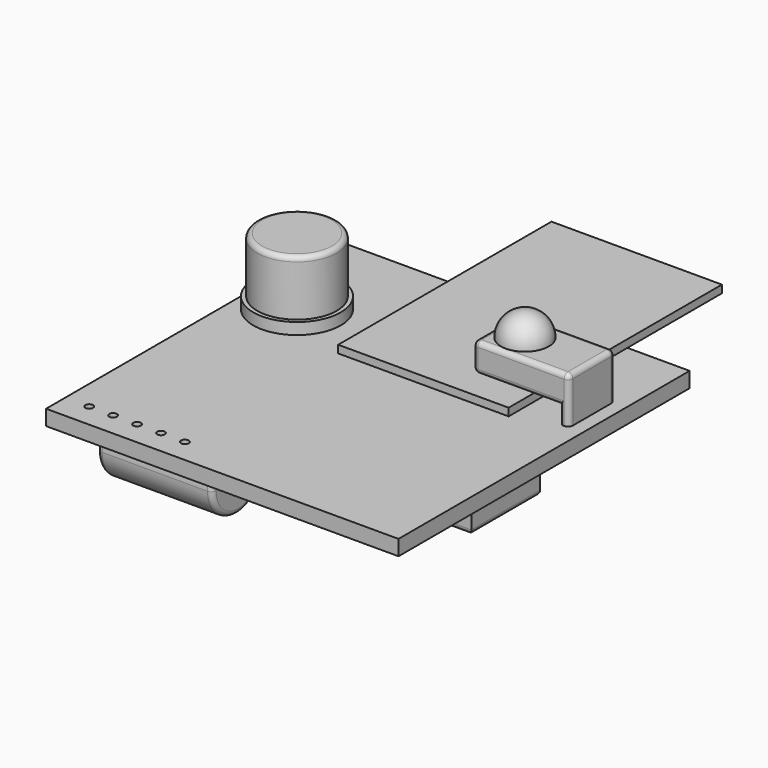
from build123d import *

# Parameters (mm, degrees)
F0_R      = 4.15
F0_W      = 10
F0_H      = 6
F1_DEPTH  = 1.6
F2_R      = 4.575
F2_R_2    = 4.15
F3_DEPTH  = 1.2
F4_R      = 4.15
F5_DEPTH  = 5.8
F2_W      = 4.9
F2_H      = 6
F2_W_2    = 17.8
F2_H_2    = 12.34
F6_DEPTH  = 0.8
F9_W      = 1
F9_H      = 6
F10_DEPTH = 1.8
F8_W      = 10
F8_H      = 6
F11_DEPTH = 3
F12_R     = 2.5
F13_DEPTH = 2.5
F14_R     = 2.49999
F15_R     = 0.49999
F16_R     = 0.4
F17_DEPTH = 25
F20_DEPTH = 12
F21_R     = 0.5
F22_W     = 18
F22_H     = 9
F23_DEPTH = 2.6
F24_R     = 0.5


# Not quite as in the source:
# - a fillet or chamfer is up to 0.001 mm smaller than in the source, because OpenCascade refuses the exact size


with BuildPart() as f1:
    # F0 (on Top) → F1 (new body)
    with BuildSketch(Plane.XY):
        Polygon((-25.5229242146, 29.8087272195), (-38.0229242146, 29.8087272195), (-38.0229242146, -8.1912727805), (-1.2229242146, -8.1912727805), (-1.2229242146, 29.8087272195), (-7.7229242146, 29.8087272195), align=None)
        with Locations((-33.0229242146, 18.3087272195)):
            Circle(F0_R, mode=Mode.SUBTRACT)
        with Locations((-7.6229242146, 18.8087272195)):
            Rectangle(F0_W, F0_H, mode=Mode.SUBTRACT)
        with Locations((-33.0229242146, 18.3087272195)):
            Circle(F0_R)
        with Locations((-7.6229242146, 18.8087272195)):
            Rectangle(F0_W, F0_H)
    extrude(amount=-F1_DEPTH)

    # F2 (on face) → F3 (join)
    with BuildSketch(Plane.XY):
        with Locations((-33.0229242146, 18.3087272195)):
            Circle(F2_R)
        with Locations((-33.0229242146, 18.3087272195)):
            Circle(F2_R_2, mode=Mode.SUBTRACT)
        with Locations((-33.0229242146, 18.3087272195)):
            Circle(F2_R_2)
    extrude(amount=F3_DEPTH)

    # F4 (on face) → F5 (join)
    with BuildSketch(Plane.XY.offset(1.2)):
        with Locations((-33.0229242146, 18.3087272195)):
            Circle(F4_R)
    extrude(amount=F5_DEPTH)

    # F2 (on face) → F6 (join)
    with BuildSketch(Plane.XY):
        with Locations((-10.1729242146, 18.8087272195)):
            Rectangle(F2_W, F2_H)
        Polygon((-7.7229242146, 15.8087272195), (-12.6229242146, 15.8087272195), (-12.6229242146, 21.8087272195), (-7.7229242146, 21.8087272195), (-7.7229242146, 29.8087272195), (-25.5229242146, 29.8087272195), (-25.5229242146, 14.3087272195), (-7.7229242146, 14.3087272195), align=None)
        with Locations((-16.6229242146, 35.9787272195)):
            Rectangle(F2_W_2, F2_H_2)
    extrude(amount=F6_DEPTH)

    # F9 (on face) → F10 (join)
    with BuildSketch(Plane.XY):
        with Locations((-3.1229242146, 18.8087272195)):
            Rectangle(F9_W, F9_H)
    extrude(amount=F10_DEPTH)

    # F8 (on offset) → F11 (join)
    with BuildSketch(Plane.XY.offset(1.8)):
        with Locations((-7.6229242146, 18.8087272195)):
            Rectangle(F8_W, F8_H)
    extrude(amount=F11_DEPTH)

    # F12 (on face) → F13 (join)
    with BuildSketch(Plane.XY.offset(4.8)):
        with Locations((-9.6229242146, 18.8087272195)):
            Circle(F12_R)
    extrude(amount=F13_DEPTH)

    # F14 (radius 2.5 in the source; OpenCascade refuses exactly that, so slightly less here)
    f14_edges = [f1.edges().sort_by_distance(p)[0] for p in [
        (-12.122924, 18.808727, 7.3),
    ]]
    fillet(f14_edges, radius=F14_R)

    # F15 (radius 0.5 in the source; OpenCascade refuses exactly that, so slightly less here)
    f15_edges = [f1.edges().sort_by_distance(p)[0] for p in [
        (-7.622924, 15.808727, 4.8),
        (-7.622924, 21.808727, 4.8),
        (-2.622924, 18.808727, 4.8),
        (-2.622924, 15.808727, 2.4),
        (-2.622924, 21.808727, 2.4),
        (-3.622924, 15.808727, 0.9),
        (-8.122924, 15.808727, 1.8),
        (-12.622924, 21.808727, 3.3),
        (-12.622924, 15.808727, 3.3),
        (-12.622924, 18.808727, 1.8),
        (-12.622924, 18.808727, 4.8),
        (-8.122924, 21.808727, 1.8),
        (-3.622924, 21.808727, 0.9),
        (-37.172924, 18.308727, 7),
    ]]
    fillet(f15_edges, radius=F15_R)

    # F16 (on face) → F17 (cut)
    with BuildSketch(Plane.XY):
        with Locations((-35.5229242146, -5.6912727805)):
            Circle(F16_R)
        with Locations((-33.0229242146, -5.6912727805)):
            Circle(F16_R)
        with Locations((-30.5229242146, -5.6912727805)):
            Circle(F16_R)
        with Locations((-28.0229242146, -5.6912727805)):
            Circle(F16_R)
        with Locations((-25.5229242146, -5.6912727805)):
            Circle(F16_R)
    extrude(amount=-F17_DEPTH, mode=Mode.SUBTRACT)

    # F19 (on offset) → F20 (join)
    with BuildSketch(Plane(origin=(-36.0229242146, 0, 0), x_dir=(0, -1, 0), z_dir=(-1, 0, 0))):
        with BuildLine():
            ThreePointArc((-0.1149529943, -1.7), (-1.3372063225, -7.5029353677), (3.9912727805, -4.9))
            ThreePointArc((3.9912727805, -4.9), (3.2942081482, -2.8715208969), (1.4974985553, -1.7))
            ThreePointArc((1.4974985553, -1.7), (1.0974747007, -1.6250954212), (0.6912727805, -1.6))
            ThreePointArc((0.6912727805, -1.6), (0.2850708603, -1.6250954212), (-0.1149529943, -1.7))
        make_face()
        with BuildLine():
            ThreePointArc((0.6912727805, -1.6), (1.0974747007, -1.6250954212), (1.4974985553, -1.7))
            Line((1.4974985553, -1.7), (1.4974985553, -1.6))
            Line((1.4974985553, -1.6), (0.6912727805, -1.6))
        make_face()
        with BuildLine():
            Line((-0.1149529943, -1.6), (-0.1149529943, -1.7))
            ThreePointArc((-0.1149529943, -1.7), (0.2850708603, -1.6250954212), (0.6912727805, -1.6))
            Line((0.6912727805, -1.6), (-0.1149529943, -1.6))
        make_face()
    extrude(amount=-F20_DEPTH)

    # F21
    f21_edges = [f1.edges().sort_by_distance(p)[0] for p in [
        (-36.022924, -0.691273, -8.2),
        (-36.022924, 0.114953, -1.65),
        (-36.022924, -1.497499, -1.65),
        (-24.022924, -1.497499, -1.65),
        (-24.022924, 0.114953, -1.65),
        (-24.022924, -0.691273, -8.2),
    ]]
    fillet(f21_edges, radius=F21_R)

    # F22 (on face) → F23 (join)
    with BuildSketch(Plane(origin=(0, 0, -1.6), x_dir=(1, 0, 0), z_dir=(0, 0, -1))):
        with Locations((-11.0229242146, -6.8087272195)):
            Rectangle(F22_W, F22_H)
    extrude(amount=F23_DEPTH)

    # F24
    f24_edges = [f1.edges().sort_by_distance(p)[0] for p in [
        (-11.022924, 2.308727, -4.2),
        (-20.022924, 6.808727, -4.2),
        (-11.022924, 11.308727, -4.2),
        (-2.022924, 6.808727, -4.2),
    ]]
    fillet(f24_edges, radius=F24_R)


solid = f1.part
